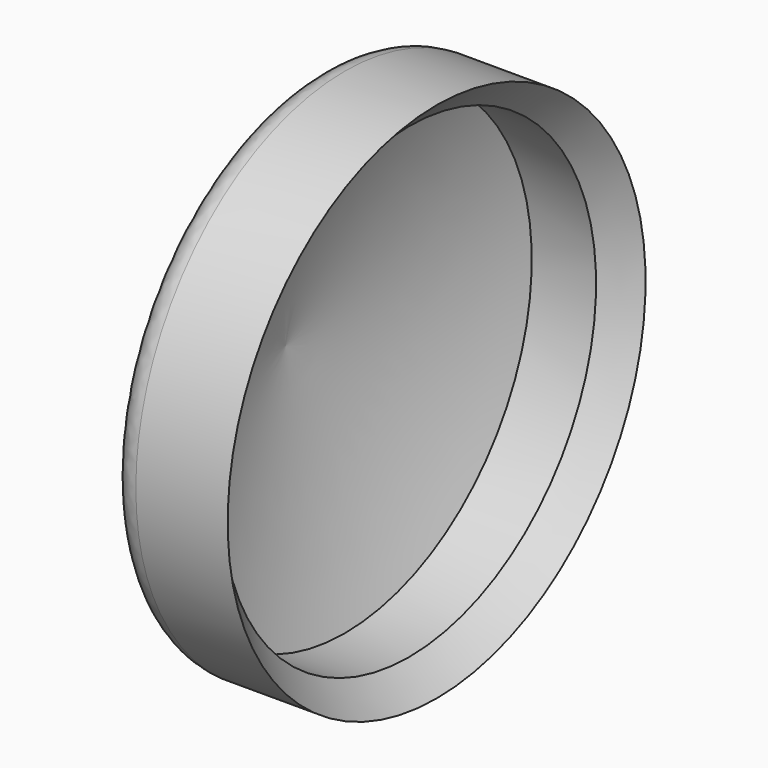
from build123d import *

# Parameters (mm, degrees)
F2_R    = 2
F3_SIZE = 1.99999


# Not quite as in the source:
# - a fillet or chamfer is up to 0.001 mm smaller than in the source, because OpenCascade refuses the exact size


with BuildPart() as f1:
    # F0 (on Front) → F1 (revolve)
    with BuildSketch(Plane.XZ):
        with BuildLine():
            Line((-13, 0), (-10.9896817121, 0))
            ThreePointArc((-10.9896817121, 0), (-9.4533501693, 8.6567410673), (-6.6803534332, 17))
            Line((-6.6803534332, 17), (0, 17))
            Line((0, 17), (0, 19))
            Line((0, 19), (-8, 19))
            ThreePointArc((-8, 19), (-11.2501561273, 9.6974095072), (-13, 0))
        make_face()
    revolve(axis=Axis((-6.5, 0, 0), (-1, 0, 0)))

    # F2
    f2_edges = [f1.edges().sort_by_distance(p)[0] for p in [
        (-8, 0, -19),
    ]]
    fillet(f2_edges, radius=F2_R)

    # F3 (size 2 in the source; OpenCascade refuses exactly that, so slightly less here)
    f3_edges = [f1.edges().sort_by_distance(p)[0] for p in [
        (0, 0, -17),
    ]]
    chamfer(f3_edges, length=F3_SIZE)


solid = f1.part
